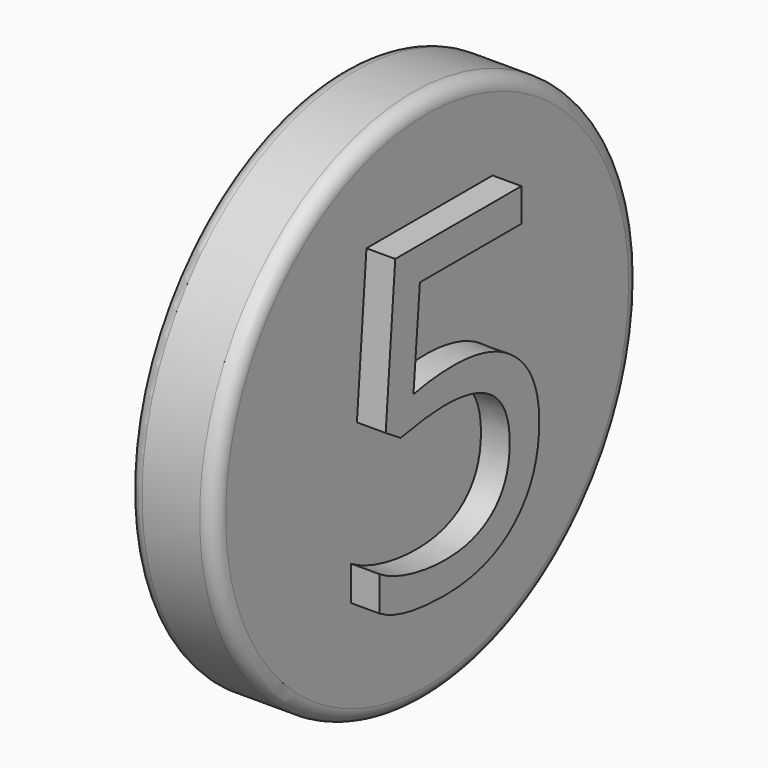
from build123d import *

# Parameters (mm, degrees)
F0_R         = 92.5
F1_DEPTH     = 30
F2_R         = 10
F3_DEPTH     = 10
F4_TEXT_SIZE = 154.2777909587
F5_DEPTH     = 10
F6_R         = 5


# Not quite as in the source:
# - Text() gives the source's letters only with a copy of the font that has no kerning and outlines rounded to 1/6400 em; it was checked with that copy


with BuildPart() as f1:
    # F0 (on Right) → F1 (new body)
    with BuildSketch(Plane.YZ):
        Circle(F0_R)
    extrude(amount=F1_DEPTH)

    # F2 (on face) → F3 (cut)
    with BuildSketch(Plane(origin=(0, 0, 0), x_dir=(0, -1, 0), z_dir=(-1, 0, 0))):
        Circle(F2_R)
    extrude(amount=-F3_DEPTH, mode=Mode.SUBTRACT)

    # F4 (on face) → F5 (join)
    with BuildSketch(Plane.YZ.offset(30)):
        with Locations((-43.1288257241, -53.0577674508)):
            Text('5', F4_TEXT_SIZE, font='Open Sans', text_align=(TextAlign.LEFT, TextAlign.BOTTOM))
    extrude(amount=F5_DEPTH)

    # F6
    f6_edges = [f1.edges().sort_by_distance(p)[0] for p in [
        (30, -92.5, 0),
        (0, -92.5, 0),
    ]]
    fillet(f6_edges, radius=F6_R)


solid = f1.part
